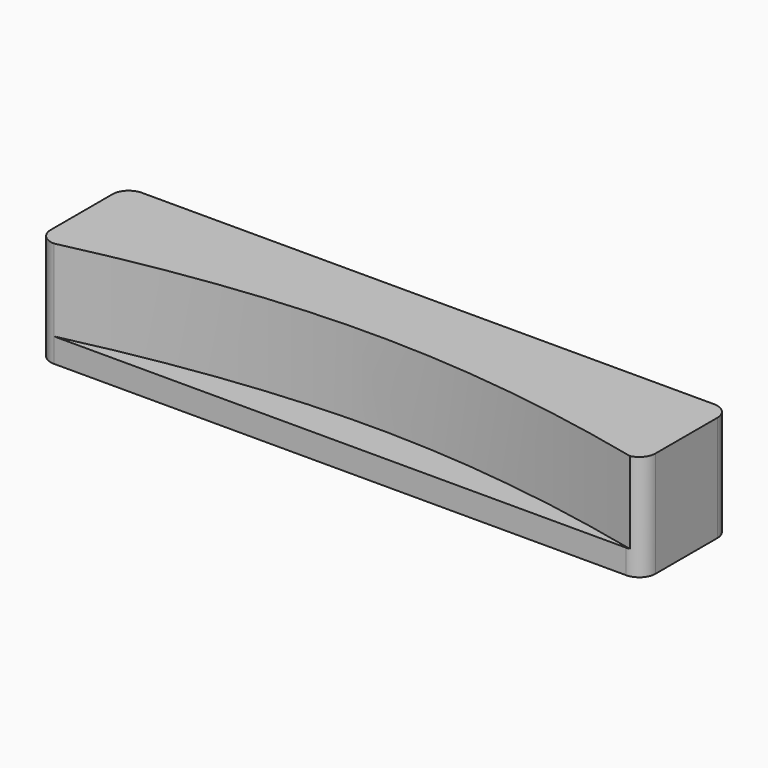
from build123d import *

# Parameters (mm, degrees)
F1_DEPTH = 32.4
F3_DEPTH = 25
F5_DEPTH = 3.2
F7_DEPTH = 20


# Not quite as in the source:
# - a feature names something its author has since deleted; it is built from what else it names


with BuildPart() as f1:
    # F0 (on Top) → F1 (new body)
    with BuildSketch(Plane.XY):
        with BuildLine():
            Line((85.6374964118, -7.5007802074), (-89.3625035882, -7.5007802074))
            ThreePointArc((-89.3625035882, -7.5007802074), (-92.8980374941, -8.9652463014), (-94.3625035882, -12.5007802074))
            Line((-94.3625035882, -12.5007802074), (-94.3625035882, -36.1007802074))
            ThreePointArc((-94.3625035882, -36.1007802074), (-92.8980374941, -39.6363141133), (-89.3625035882, -41.1007802074))
            add(Edge.make_bspline(
                [(-89.3625035882, -41.1007802074), (-59.4132024584, -34.6381396439), (-0.1322912347, -21.8461476087), (57.2468589299, -34.7273087443), (85.6374964118, -41.1007802074)],
                knots=[0, 0, 0, 0, 0.5052098646, 1, 1, 1, 1], degree=3))
            ThreePointArc((85.6374964118, -41.1007802074), (89.1730303177, -39.6363141133), (90.6374964118, -36.1007802074))
            Line((90.6374964118, -36.1007802074), (90.6374964118, -12.5007802074))
            ThreePointArc((90.6374964118, -12.5007802074), (89.1730303177, -8.9652463014), (85.6374964118, -7.5007802074))
        make_face()
        with BuildLine():
            add(Edge.make_bspline(
                [(-89.3625035882, -41.1007802074), (-59.4132024584, -34.6381396439), (-0.1322912347, -21.8461476087), (57.2468589299, -34.7273087443), (85.6374964118, -41.1007802074)],
                knots=[0, 0, 0, 0, 0.5052098646, 1, 1, 1, 1], degree=3))
            Line((-89.3625035882, -41.1007802074), (85.6374964118, -41.1007802074))
        make_face()
    extrude(amount=F1_DEPTH)

    # F2 (on face) → F3 (cut)
    with BuildSketch(Plane.XY.offset(32.4)):
        with BuildLine():
            add(Edge.make_bspline(
                [(-89.3625035882, -41.1007802074), (-59.456438476, -34.254019451), (-0.1066600814, -25.9658719218), (57.8851377231, -34.2465879534), (86.657191818, -40.9956981105)],
                knots=[0, 0, 0, 0, 0.5038023595, 1, 1, 1, 1], degree=3))
            Line((-89.3625035882, -41.1007802074), (85.6374964118, -41.1007802074))
            ThreePointArc((85.6374964118, -41.1007802074), (86.1500442068, -41.0744403041), (86.657191818, -40.9956981105))
        make_face()
    extrude(amount=-F3_DEPTH, mode=Mode.SUBTRACT)

    # F4 (on face) → F5 (join)
    with BuildSketch(Plane(origin=(0, 0, 0), x_dir=(1, 0, 0), z_dir=(0, 0, -1))):
        with BuildLine():
            Line((-51.5625035882, 18.8695881516), (-54.9125035882, 18.8695881516))
            ThreePointArc((-54.9125035882, 18.8695881516), (-51.5625035882, 15.5195881516), (-48.2125035882, 18.8695881516))
            Line((-48.2125035882, 18.8695881516), (-51.5625035882, 18.8695881516))
        make_face()
        with BuildLine():
            ThreePointArc((-48.2125035882, 18.8695881516), (-51.5625035882, 22.2195881516), (-54.9125035882, 18.8695881516))
            Line((-54.9125035882, 18.8695881516), (-51.5625035882, 18.8695881516))
            Line((-51.5625035882, 18.8695881516), (-48.2125035882, 18.8695881516))
        make_face()
        with BuildLine():
            ThreePointArc((51.1874964118, 18.8695881516), (47.8374964118, 22.2195881516), (44.4874964118, 18.8695881516))
            Line((44.4874964118, 18.8695881516), (47.8374964118, 18.8695881516))
            Line((47.8374964118, 18.8695881516), (51.1874964118, 18.8695881516))
        make_face()
        with BuildLine():
            Line((47.8374964118, 18.8695881516), (44.4874964118, 18.8695881516))
            ThreePointArc((44.4874964118, 18.8695881516), (47.8374964118, 15.5195881516), (51.1874964118, 18.8695881516))
            Line((51.1874964118, 18.8695881516), (47.8374964118, 18.8695881516))
        make_face()
    extrude(amount=F5_DEPTH)

    # F6 (on face) → F7 (cut)
    with BuildSketch(Plane(origin=(0, 0, -3.2), x_dir=(1, 0, 0), z_dir=(0, 0, -1))):
        with BuildLine():
            ThreePointArc((49.7674964118, 18.8695881516), (46.6597964296, 20.3986148851), (47.3447785341, 17.0035417714))
            ThreePointArc((47.3447785341, 17.0035417714), (49.015196394, 17.340561418), (49.7674964118, 18.8695881516))
        make_face()
        with BuildLine():
            ThreePointArc((-52.6547781922, 17.2789104499), (-50.6630550607, 17.1616089388), (-49.6317802739, 18.8695881516))
            ThreePointArc((-49.6317802739, 18.8695881516), (-52.4605054871, 20.5775673643), (-52.6547781922, 17.2789104499))
        make_face()
    extrude(amount=-F7_DEPTH, mode=Mode.SUBTRACT)


solid = f1.part
